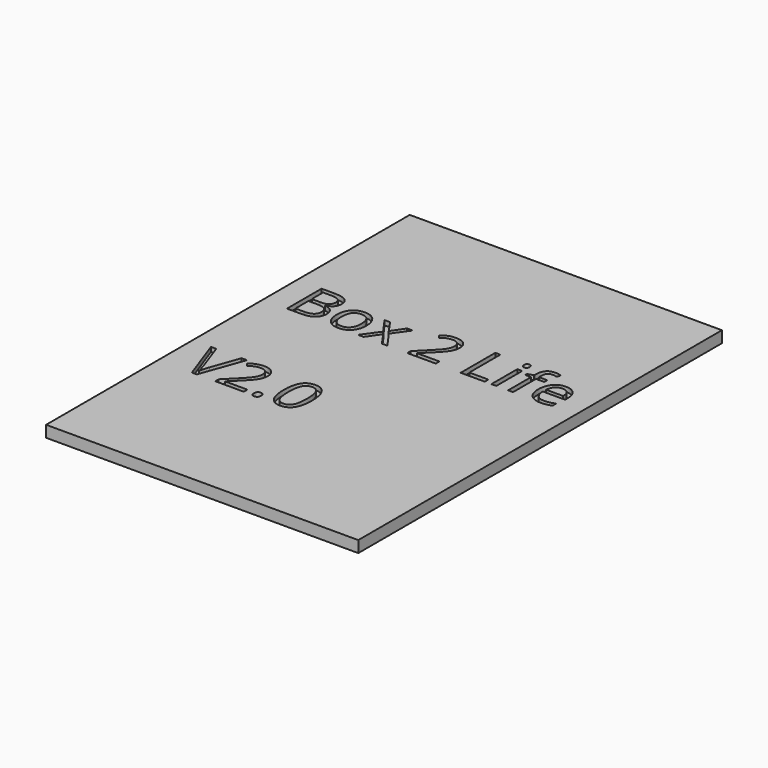
from build123d import *

# Parameters (mm, degrees)
F0_W         = 68
F0_H         = 99
F1_DEPTH     = 2.5
F2_TEXT_SIZE = 13.1944444444
F3_DEPTH     = 1


# Not quite as in the source:
# - Text() gives the source's letters only with a copy of the font that has no kerning and outlines rounded to 1/6400 em; it was checked with that copy


with BuildPart() as f1:
    # F0 (on Top) → F1 (new body)
    with BuildSketch(Plane.XY):
        with Locations((34, 49.5)):
            Rectangle(F0_W, F0_H)
    extrude(amount=F1_DEPTH)

    # F2 (on face) → F3 (cut)
    with BuildSketch(Plane.XY.offset(2.5)):
        with Locations((3.9702690972, 59)):
            Text('Box 2 Life', F2_TEXT_SIZE, font='Open Sans', text_align=(TextAlign.LEFT, TextAlign.BOTTOM))
        with Locations((3.9702690972, 30.5)):
            Text('V2.0', F2_TEXT_SIZE, font='Open Sans', text_align=(TextAlign.LEFT, TextAlign.BOTTOM))
    extrude(amount=-F3_DEPTH, mode=Mode.SUBTRACT)


solid = f1.part
